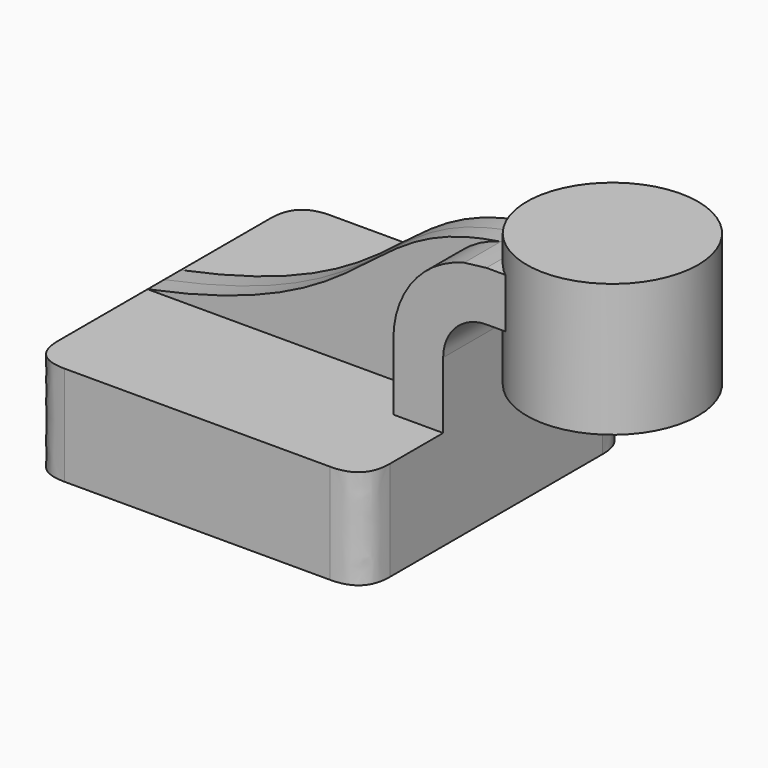
from build123d import *

# Parameters (mm, degrees)
F1_DEPTH    = 63.5
F2_DEPTH    = 25.4
F3_DEPTH    = 7.9375
F5_T1_DEPTH = 101.6


# Not quite as in the source:
# - a fillet or chamfer that OpenCascade refuses, or shapes differently, is made with other operations: its cross-section is extruded or revolved along the edge and cut away or added


with BuildPart() as f1:
    # F0 (on Front) → F1 (new body, symmetric)
    with BuildSketch(Plane.XZ):
        Polygon((44.45, 19.05), (-63.5, 19.05), (-63.5, -19.05), (63.5, -19.05), (63.5, 19.05), align=None)
    extrude(amount=F1_DEPTH, both=True)

    # F0 (on Front) → F2 (join, symmetric)
    with BuildSketch(Plane.XZ):
        with BuildLine():
            Line((44.45, 44.45), (44.45, 19.05))
            Line((44.45, 19.05), (63.5, 19.05))
            Line((63.5, 19.05), (63.5, 44.45))
            ThreePointArc((63.5, 44.45), (68.3356670426, 56.1243329574), (80.01, 60.96))
            Line((80.01, 60.96), (89.8442984975, 60.96))
            Line((89.8442984975, 60.96), (89.8442984975, 80.01))
            Line((89.8442984975, 80.01), (80.01, 80.01))
            add(Edge.make_bspline(
                [(71.5290560563, 78.9838557046), (74.194576587, 79.3820969631), (77.0154135084, 79.7255153509), (80.01, 80.01)],
                knots=[148.8797919707, 148.8797919707, 148.8797919707, 148.8797919707, 155.9206262815, 155.9206262815, 155.9206262815, 155.9206262815], degree=3))
            ThreePointArc((71.5290560563, 78.9838557046), (52.0270054619, 66.3923247784), (44.45, 44.45))
        make_face()
    extrude(amount=F2_DEPTH, both=True)

    # F0 (on Front) → F3 (join, symmetric)
    with BuildSketch(Plane.XZ):
        with BuildLine():
            add(Edge.make_bspline(
                [(-63.5, 19.05), (28.2481007656, 37.6297254633), (15.1661131725, 70.5629679071), (71.5290560563, 78.9838557046)],
                knots=[0, 0, 0, 0, 148.8797919707, 148.8797919707, 148.8797919707, 148.8797919707], degree=3))
            Line((-63.5, 19.05), (44.45, 19.05))
            Line((44.45, 19.05), (44.45, 44.45))
            ThreePointArc((44.45, 44.45), (52.0270054619, 66.3923247784), (71.5290560563, 78.9838557046))
        make_face()
    extrude(amount=F3_DEPTH, both=True)

    # F5: fillet of radius 12.7 on 4 edges, made by hand

    # F5_s2 → F5_t1 (cut)
    with BuildSketch(Plane.XY.offset(-50.8)):
        with BuildLine():
            add(Edge.make_bspline(
                [(-63.5, -50.8), (-63.5, -63.5), (-50.8, -63.5)],
                knots=[0, 0, 0, 1, 1, 1], degree=2, weights=[1, 1, 1]))
            Line((-50.8, -63.5), (-63.5, -63.5))
            Line((-63.5, -63.5), (-63.5, -50.8))
        make_face()
        with BuildLine():
            add(Edge.make_bspline(
                [(63.5, -50.8), (63.5, -63.5), (50.8, -63.5)],
                knots=[0, 0, 0, 1, 1, 1], degree=2, weights=[1, 1, 1]))
            Line((50.8, -63.5), (63.5, -63.5))
            Line((63.5, -63.5), (63.5, -50.8))
        make_face()
        with BuildLine():
            add(Edge.make_bspline(
                [(63.5, 50.8), (63.5, 63.5), (50.8, 63.5)],
                knots=[0, 0, 0, 1, 1, 1], degree=2, weights=[1, 1, 1]))
            Line((50.8, 63.5), (63.5, 63.5))
            Line((63.5, 63.5), (63.5, 50.8))
        make_face()
        with BuildLine():
            add(Edge.make_bspline(
                [(-63.5, 50.8), (-63.5, 63.5), (-50.8, 63.5)],
                knots=[0, 0, 0, 1, 1, 1], degree=2, weights=[1, 1, 1]))
            Line((-50.8, 63.5), (-63.5, 63.5))
            Line((-63.5, 63.5), (-63.5, 50.8))
        make_face()
    extrude(amount=F5_T1_DEPTH, mode=Mode.SUBTRACT)


with BuildPart() as f4:
    # F0 (on Front) → F4 (revolve)
    with BuildSketch(Plane.XZ):
        Polygon((107.8898191703, 90.4005332853), (107.8898191703, 80.01), (107.8898191703, 60.96), (107.8898191703, 39.6005332853), (140.6442984975, 39.6005332853), (140.6442984975, 90.4005332853), align=None)
    revolve(axis=Axis((107.8898191703, 0, 65.0005332853), (0, 0, 1)))


solid = Compound([f1.part, f4.part])
